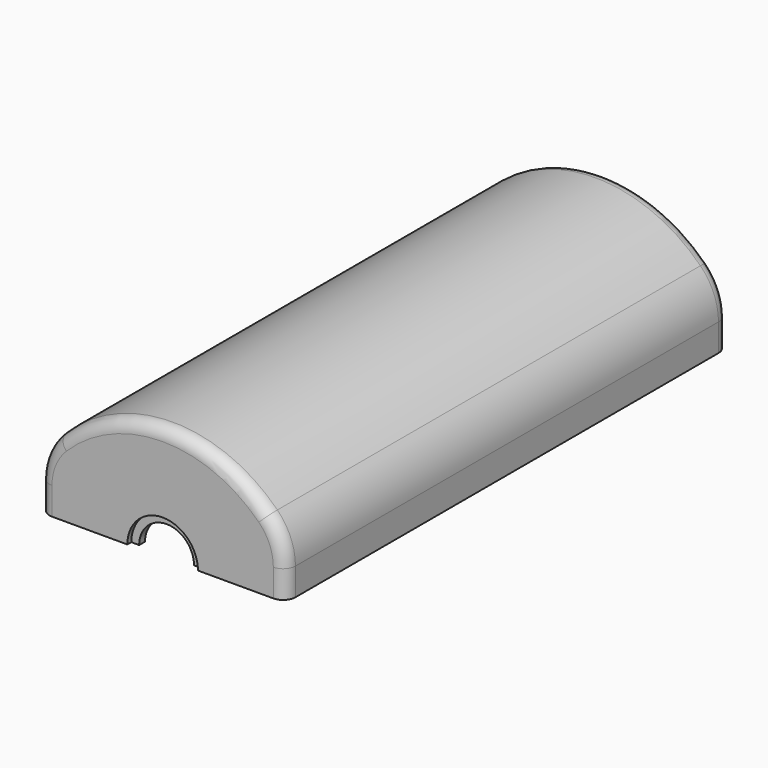
from build123d import *

# Parameters (mm, degrees)
F0_W      = 20
F0_H      = 4
F1_DEPTH  = 45
F2_T      = -1
F3_R      = 5
F4_R      = 5
F6_DEPTH  = 3
F7_R      = 0.7
F8_DEPTH  = 3
F9_R      = 1
F10_R     = 1
F12_DEPTH = 50
F13_DEPTH = 0.4
F15_DEPTH = 0.4


with BuildPart() as f1:
    # F0 (on Front) → F1 (new body)
    with BuildSketch(Plane.XZ):
        with Locations((10, 2)):
            Rectangle(F0_W, F0_H)
        with BuildLine():
            ThreePointArc((20, 4), (10, 9.301808562), (0, 4))
            Line((0, 4), (20, 4))
        make_face()
    extrude(amount=F1_DEPTH)

    # F2
    f2_openings = [f1.faces().sort_by_distance(p)[0] for p in [
        (10, -22.5, 0),
    ]]
    offset(amount=F2_T, openings=f2_openings)

    # F3
    f3_edges = [f1.edges().sort_by_distance(p)[0] for p in [
        (0, -22.5, 4),
    ]]
    fillet(f3_edges, radius=F3_R)

    # F4
    f4_edges = [f1.edges().sort_by_distance(p)[0] for p in [
        (20, -22.5, 4),
    ]]
    fillet(f4_edges, radius=F4_R)

    # F5 (on face) → F6 (join)
    with BuildSketch(Plane(origin=(0, 0, 0), x_dir=(1, 0, 0), z_dir=(0, 0, -1))):
        with BuildLine():
            Line((1, 1), (1.9, 1))
            ThreePointArc((1.9, 1), (1.6363961031, 1.6363961031), (1, 1.9))
            Line((1, 1.9), (1, 1))
        make_face()
        with BuildLine():
            ThreePointArc((19, 1.9), (18.3636038969, 1.6363961031), (18.1, 1))
            Line((18.1, 1), (19, 1))
            Line((19, 1), (19, 1.9))
        make_face()
        with BuildLine():
            ThreePointArc((18.1, 44), (18.3636038969, 43.3636038969), (19, 43.1))
            Line((19, 43.1), (19, 44))
            Line((19, 44), (18.1, 44))
        make_face()
        with BuildLine():
            Line((1, 44), (1, 43.1))
            ThreePointArc((1, 43.1), (1.6363961031, 43.3636038969), (1.9, 44))
            Line((1.9, 44), (1, 44))
        make_face()
    extrude(amount=-F6_DEPTH)

    # F7 (on face) → F8 (cut)
    with BuildSketch(Plane(origin=(0, 0, 0), x_dir=(1, 0, 0), z_dir=(0, 0, -1))):
        with Locations((1, 1)):
            Circle(F7_R)
        with Locations((19, 1)):
            Circle(F7_R)
        with Locations((1, 44)):
            Circle(F7_R)
        with Locations((19, 44)):
            Circle(F7_R)
    extrude(amount=-F8_DEPTH, mode=Mode.SUBTRACT)

    # F9
    f9_edges = [f1.edges().sort_by_distance(p)[0] for p in [
        (20, -45, 1.117556),
        (19.617968, -45, 4.151977),
        (10, -45, 9.301809),
        (0.382032, -45, 4.151977),
        (0, -45, 1.117556),
    ]]
    fillet(f9_edges, radius=F9_R)

    # F10
    f10_edges = [f1.edges().sort_by_distance(p)[0] for p in [
        (0, 0, 1.117556),
        (0.382032, 0, 4.151977),
        (10, 0, 9.301809),
        (19.617968, 0, 4.151977),
        (20, 0, 1.117556),
    ]]
    fillet(f10_edges, radius=F10_R)

    # F11 (on face) → F12 (cut)
    with BuildSketch(Plane.XZ.offset(45)):
        with BuildLine():
            Line((7.7686794017, 0), (12.2313205983, 0))
            ThreePointArc((12.2313205983, 0), (10, 2.2313205983), (7.7686794017, 0))
        make_face()
    extrude(amount=-F12_DEPTH, mode=Mode.SUBTRACT)

    # F11 (on face) → F13 (cut)
    with BuildSketch(Plane.XZ.offset(45)):
        with BuildLine():
            Line((12.2313205983, 0), (12.8707642747, 0))
            ThreePointArc((12.8707642747, 0), (10, 2.8707642747), (7.1292357253, 0))
            Line((7.1292357253, 0), (7.7686794017, 0))
            ThreePointArc((7.7686794017, 0), (10, 2.2313205983), (12.2313205983, 0))
        make_face()
    extrude(amount=-F13_DEPTH, mode=Mode.SUBTRACT)

    # F14 (on face) → F15 (cut)
    with BuildSketch(Plane(origin=(0, 0, 0), x_dir=(-1, 0, 0), z_dir=(0, 1, 0))):
        with BuildLine():
            Line((-7.7686794017, 0), (-7.1292357253, 0))
            ThreePointArc((-7.1292357253, 0), (-10, 2.8707642747), (-12.8707642747, 0))
            Line((-12.8707642747, 0), (-12.2313205983, 0))
            ThreePointArc((-12.2313205983, 0), (-10, 2.2313205983), (-7.7686794017, 0))
        make_face()
    extrude(amount=-F15_DEPTH, mode=Mode.SUBTRACT)


solid = f1.part
